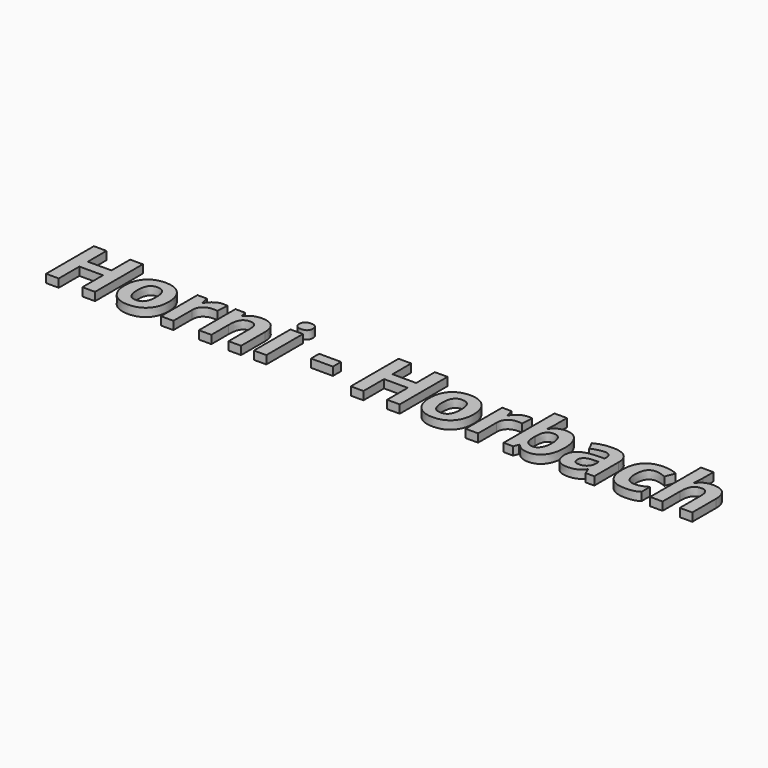
from build123d import *

# Parameters (mm, degrees)
F0_TEXT_SIZE = 30.4539403361
F1_DEPTH     = 3


# Not quite as in the source:
# - Text() gives the source's letters only with a copy of the font that has no kerning and outlines rounded to 1/6400 em; it was checked with that copy


with BuildPart() as f1:
    # F0 (on Top) → F1 (new body)
    with BuildSketch(Plane.XY):
        with Locations((0, 0)):
            Text('Horni - Horbach', F0_TEXT_SIZE, font='Open Sans', font_style=FontStyle.BOLD, text_align=(TextAlign.LEFT, TextAlign.BOTTOM))
    extrude(amount=F1_DEPTH)


solid = f1.part
